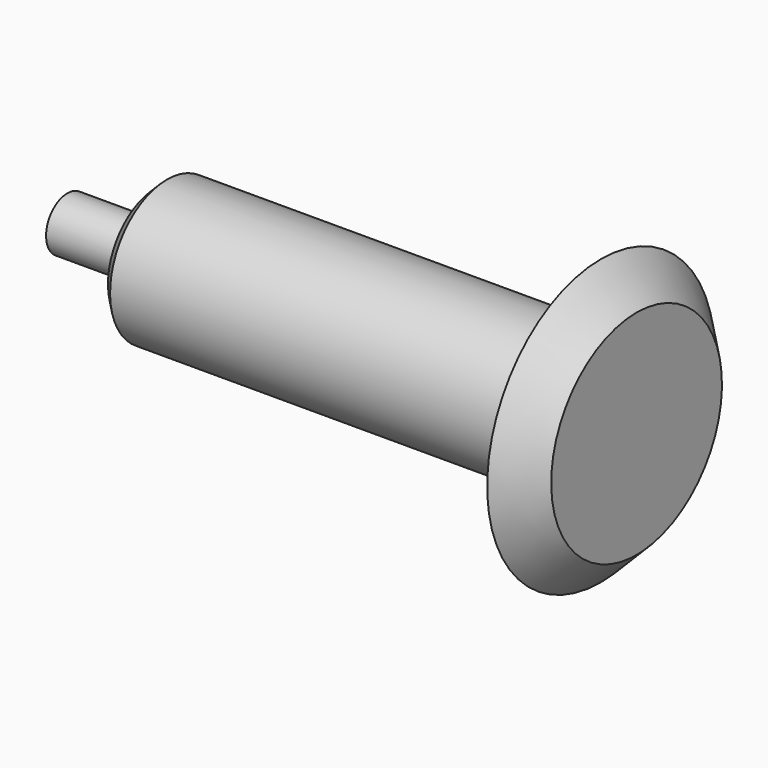
from build123d import *

# Parameters (mm, degrees)
F2_SIZE = 9.99999
F3_SIZE = 10
F4_SIZE = 3


# Not quite as in the source:
# - a fillet or chamfer is up to 0.001 mm smaller than in the source, because OpenCascade refuses the exact size


with BuildPart() as f1:
    # F0 (on Front) → F1 (revolve)
    with BuildSketch(Plane.XZ):
        Polygon((0, 0), (0, 40), (-10, 40), (-10, 20), (-135, 20), (-135, 7.5), (-160, 7.5), (-160, 0), align=None)
    revolve(axis=Axis((-80, 0, 0), (1, 0, 0)))

    # F2 (size 10 in the source; OpenCascade refuses exactly that, so slightly less here)
    f2_edges = [f1.edges().sort_by_distance(p)[0] for p in [
        (0, 0, -40),
    ]]
    chamfer(f2_edges, length=F2_SIZE)

    # F3
    f3_edges = [f1.edges().sort_by_distance(p)[0] for p in [
        (-10, 0, -20),
    ]]
    chamfer(f3_edges, length=F3_SIZE)

    # F4
    f4_edges = [f1.edges().sort_by_distance(p)[0] for p in [
        (-135, 0, -20),
    ]]
    chamfer(f4_edges, length=F4_SIZE)


solid = f1.part
